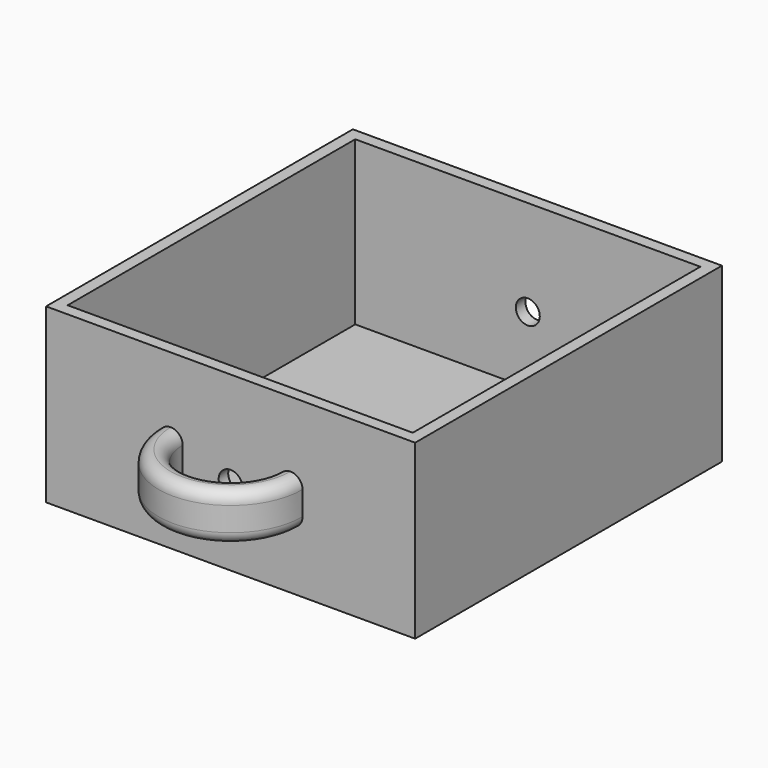
from build123d import *

# Parameters (mm, degrees)
F0_W      = 97.79
F0_H      = 45.72
F1_DEPTH  = 101.6
F2_W      = 91.44
F2_H      = 95.25
F3_DEPTH  = 43.18
F4_W      = 19.05
F4_H      = 6.35
F5_ANGLE  = 180
F7_DEPTH  = 25.4
F8_R      = 3.17499
F10_D     = 6.35
F10_DEPTH = 101.601


# Not quite as in the source:
# - a fillet or chamfer is up to 0.001 mm smaller than in the source, because OpenCascade refuses the exact size


with BuildPart() as f1:
    # F0 (on Front) → F1 (new body)
    with BuildSketch(Plane.XZ):
        with Locations((15.4838143581, 4.6649015626)):
            Rectangle(F0_W, F0_H)
    extrude(amount=-F1_DEPTH)

    # F2 (on face) → F3 (cut)
    with BuildSketch(Plane.XY.offset(27.5249015626)):
        with Locations((15.4838143581, 50.8)):
            Rectangle(F2_W, F2_H)
    extrude(amount=-F3_DEPTH, mode=Mode.SUBTRACT)

    # F4 (on face) → F5 (revolve)
    with BuildSketch(Plane.XZ):
        with Locations((5.9588143581, 6.8874015626)):
            Rectangle(F4_W, F4_H)
        with Locations((5.9588143581, 0.5374015626)):
            Rectangle(F4_W, F4_H)
    revolve(axis=Axis((15.4838143581, 0, 3.7124015626), (0, 0, 1)), revolution_arc=F5_ANGLE)

    # F6 (on face) → F7 (cut)
    with BuildSketch(Plane.XY.offset(10.0624015626)):
        with BuildLine():
            Line((28.1838143581, 0), (2.7838143581, 0))
            ThreePointArc((2.7838143581, 0), (15.4838143581, -12.7), (28.1838143581, 0))
        make_face()
    extrude(amount=-F7_DEPTH, mode=Mode.SUBTRACT)

    # F8 (radius 3.175 in the source; OpenCascade refuses exactly that, so slightly less here)
    f8_edges = [f1.edges().sort_by_distance(p)[0] for p in [
        (15.483814, -19.05, 10.062402),
        (15.483814, -12.7, 10.062402),
        (15.483814, -19.05, -2.637598),
        (15.483814, -12.7, -2.637598),
    ]]
    fillet(f8_edges, radius=F8_R)

    # F10 (through all, one way)
    with BuildSketch(Plane.XZ):
        with Locations((15.4838143581, 2.1249015626)):
            Circle(F10_D / 2)
    extrude(amount=-F10_DEPTH, mode=Mode.SUBTRACT)


solid = f1.part
